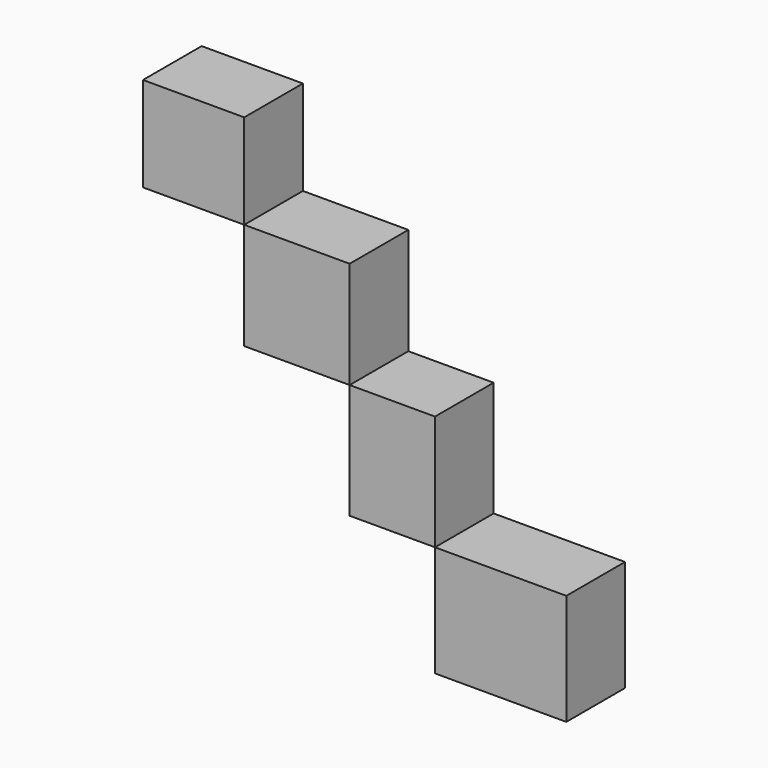
from build123d import *

# Parameters (mm, degrees)
F0_W     = 45.4829260707
F0_H     = 38.4368486702
F1_DEPTH = 25.4
F0_W_2   = 29.5494180173
F0_H_2   = 39.8497525603
F0_W_3   = 36.5022253245
F0_H_3   = 36.9735397398
F0_W_4   = 35.0537188351
F0_H_4   = 32.7565018088


# Not quite as in the source:
# - a feature of the source that left no trace in its solid (it failed there, or was rolled back) is left out


with BuildPart() as f1:
    # F0 (on Front) → F1 (new body)
    with BuildSketch(Plane.XZ):
        with Locations((44.4689802825, -76.1008691043)):
            Rectangle(F0_W, F0_H)
    extrude(amount=F1_DEPTH)


with BuildPart() as f1b:
    # F0 (on Front) → F1, piece 2 (new body)
    with BuildSketch(Plane.XZ):
        with Locations((6.9528082386, -36.957568489)):
            Rectangle(F0_W_2, F0_H_2)
    extrude(amount=F1_DEPTH)


with BuildPart() as f1c:
    # F0 (on Front) → F1, piece 3 (new body)
    with BuildSketch(Plane.XZ):
        with Locations((-26.0730134323, 1.454077661)):
            Rectangle(F0_W_3, F0_H_3)
    extrude(amount=F1_DEPTH)


with BuildPart() as f1d:
    # F0 (on Front) → F1, piece 4 (new body)
    with BuildSketch(Plane.XZ):
        with Locations((-61.8509855121, 36.3190984353)):
            Rectangle(F0_W_4, F0_H_4)
    extrude(amount=F1_DEPTH)


solid = Compound([f1.part, f1b.part, f1c.part, f1d.part])
